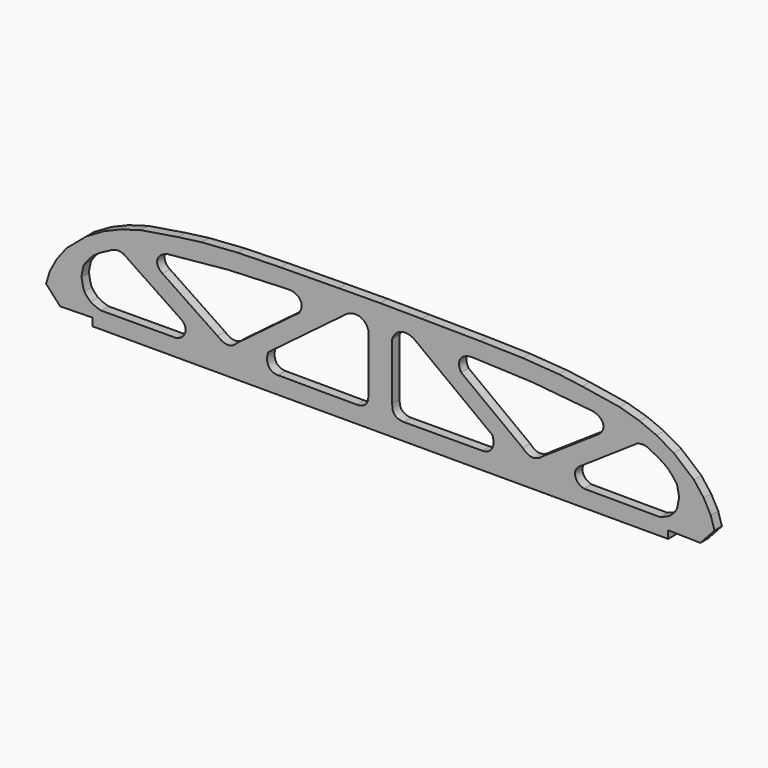
from build123d import *

# Parameters (mm, degrees)
F1_DEPTH = 3


# Not quite as in the source:
# - ends of sketch curves that miss each other by under 0.0002 mm in the source are joined


with BuildPart() as f1:
    # F0 (on Front) → F1 (new body)
    with BuildSketch(Plane.XZ):
        Polygon((-0.0539638903, 18.370702), (-0.0038508903, -18.362152), (92.7633391097, -18.370702), (92.6924631097, -15.890233), (103.1813041097, -16.102845), (107.7170111097, -11.141907), (106.5122111097, -7.173158), (104.2443611097, -2.991796), (101.0845361097, 1.130854), (94.6101381097, 6.599435), (89.0528781097, 9.821526), (83.6210411097, 12.103627), (77.1418581097, 13.991338), (65.1238321097, 15.930635), (57.6115531097, 16.922822), (45.9973841097, 17.743913), (32.1186031097, 18.070024), (13.3763291097, 18.270477), align=None)
        with BuildLine():
            add(Edge.make_bspline(
                [(65.6943371097, -12.899831), (62.5550341097, -12.172951), (61.7713101097, -8.692501), (64.1909471097, -7.08672)],
                knots=[0, 0, 0, 0, 1, 1, 1, 1], degree=3))
            Line((64.1909471097, -7.08672), (82.7828791097, 5.441539))
            add(Edge.make_bspline(
                [(82.7828791097, 5.441539), (83.8783131097, 5.841711), (85.0121781097, 5.972881), (86.2406861097, 5.441541)],
                knots=[0, 0, 0, 0, 1, 1, 1, 1], degree=3))
            add(Edge.make_bspline(
                [(86.2406861097, 5.441541), (88.5854111097, 4.25464), (90.9595961097, 3.079519), (92.6551511097, 1.632949)],
                knots=[0, 0, 0, 0, 1, 1, 1, 1], degree=3))
            add(Edge.make_bspline(
                [(92.6551511097, 1.632949), (93.7989981097, 0.505006), (94.7332961097, -0.581922), (95.6118231097, -1.97519)],
                knots=[0, 0, 0, 0, 1, 1, 1, 1], degree=3))
            add(Edge.make_bspline(
                [(95.6118231097, -1.97519), (95.8557461097, -3.177903), (96.2772981097, -4.480841), (96.2632881097, -5.683554)],
                knots=[0, 0, 0, 0, 1, 1, 1, 1], degree=3))
            add(Edge.make_bspline(
                [(96.2632881097, -5.683554), (95.9762411097, -6.899896), (95.9073311097, -8.384491), (95.3612561097, -9.341805)],
                knots=[0, 0, 0, 0, 1, 1, 1, 1], degree=3))
            add(Edge.make_bspline(
                [(95.3612561097, -9.341805), (94.8500481097, -10.267174), (94.1296281097, -10.933218), (93.3567311097, -11.596892)],
                knots=[0, 0, 0, 0, 1, 1, 1, 1], degree=3))
            add(Edge.make_bspline(
                [(93.3567311097, -11.596892), (92.4958131097, -12.139141), (91.1271531097, -12.72489), (89.9991611097, -13.000059)],
                knots=[0, 0, 0, 0, 1, 1, 1, 1], degree=3))
            Line((89.9991611097, -13.000059), (65.6943371097, -12.899831))
        make_face(mode=Mode.SUBTRACT)
        with BuildLine():
            Line((3.8548531097, -8.790562), (3.8548531097, 9.450582))
            add(Edge.make_bspline(
                [(10.8706771097, 11.755782), (8.5680291097, 13.13931), (5.1563371097, 13.150107), (3.8548531097, 9.450582)],
                knots=[0, 0, 0, 0, 1, 1, 1, 1], degree=3))
            Line((10.8706771097, 11.755782), (36.1276481097, -7.28717))
            add(Edge.make_bspline(
                [(32.9204121097, -12.799606), (35.7071221097, -12.751328), (37.1961481097, -10.572453), (36.1276481097, -7.28717)],
                knots=[0, 0, 0, 0, 1, 1, 1, 1], degree=3))
            Line((32.9204121097, -12.799606), (7.5632171097, -12.899831))
            add(Edge.make_bspline(
                [(3.8548531097, -8.790562), (3.7573371097, -11.04941), (4.4717691097, -12.766958), (7.5632171097, -12.899831)],
                knots=[0, 0, 0, 0, 1, 1, 1, 1], degree=3))
        make_face(mode=Mode.SUBTRACT)
        with BuildLine():
            Line((45.9498021097, -7.788301), (26.1050401097, 7.145382))
            add(Edge.make_bspline(
                [(29.7131791097, 12.657816), (26.6289141097, 12.752098), (24.0319891097, 10.480568), (26.1050401097, 7.145382)],
                knots=[0, 0, 0, 0, 1, 1, 1, 1], degree=3))
            Line((29.7131791097, 12.657816), (49.0586381097, 11.882658))
            Line((49.0586381097, 11.882658), (68.4505551097, 10.001826))
            add(Edge.make_bspline(
                [(70.2045121097, 3.938149), (72.7849811097, 5.68209), (72.6619441097, 8.999483), (68.4505551097, 10.001826)],
                knots=[0, 0, 0, 0, 1, 1, 1, 1], degree=3))
            Line((70.2045121097, 3.938149), (52.4644981097, -7.988753))
            add(Edge.make_bspline(
                [(45.9498021097, -7.788301), (47.6692371097, -9.607126), (49.6811001097, -10.292787), (52.4644981097, -7.988753)],
                knots=[0, 0, 0, 0, 1, 1, 1, 1], degree=3))
        make_face(mode=Mode.SUBTRACT)
    extrude(amount=F1_DEPTH)

    # F2: F1 across plane


with BuildPart() as f1_1:
    add(f1.part)
    add(f1.part.mirror(Plane.YZ))


solid = f1_1.part
